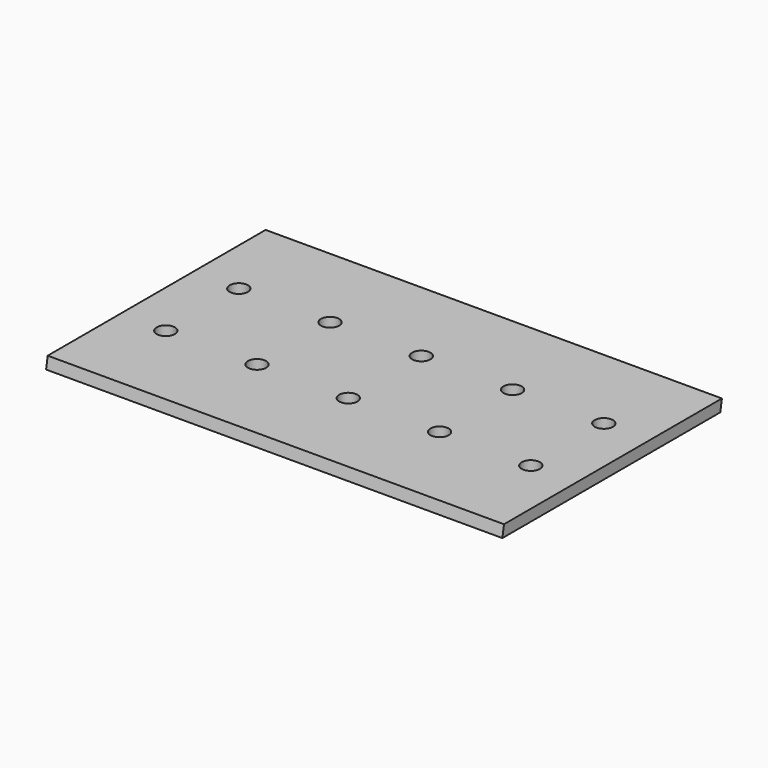
from build123d import *

# Parameters (mm, degrees)
F0_W     = 254
F0_H     = 165.1
F0_R     = 5.08
F1_DEPTH = 6.35
F3_DEPTH = 254.001
F5_DEPTH = 254.001


with BuildPart() as f1:
    # F0 (on Top) → F1 (new body)
    with BuildSketch(Plane.XY):
        with Locations((127, 82.55)):
            Rectangle(F0_W, F0_H)
        with Locations((25.4, 63.881)):
            Circle(F0_R, mode=Mode.SUBTRACT)
        with Locations((76.2, 63.881)):
            Circle(F0_R, mode=Mode.SUBTRACT)
        with Locations((127, 63.881)):
            Circle(F0_R, mode=Mode.SUBTRACT)
        with Locations((177.8, 63.881)):
            Circle(F0_R, mode=Mode.SUBTRACT)
        with Locations((228.6, 63.881)):
            Circle(F0_R, mode=Mode.SUBTRACT)
        with Locations((25.4, 114.681)):
            Circle(F0_R, mode=Mode.SUBTRACT)
        with Locations((76.2, 114.681)):
            Circle(F0_R, mode=Mode.SUBTRACT)
        with Locations((127, 114.681)):
            Circle(F0_R, mode=Mode.SUBTRACT)
        with Locations((177.8, 114.681)):
            Circle(F0_R, mode=Mode.SUBTRACT)
        with Locations((228.6, 114.681)):
            Circle(F0_R, mode=Mode.SUBTRACT)
    extrude(amount=F1_DEPTH)

    # F2 (on face) → F3 (cut, through all)
    with BuildSketch(Plane(origin=(0, 0, 0), x_dir=(0, -1, 0), z_dir=(-1, 0, 0))):
        Polygon((-163.9803236725, 0), (-165.1, 6.35), (-165.1, 0), align=None)
    extrude(amount=-F3_DEPTH, mode=Mode.SUBTRACT)

    # F4 (on face) → F5 (cut, through all)
    with BuildSketch(Plane(origin=(0, 0, 0), x_dir=(0, -1, 0), z_dir=(-1, 0, 0))):
        Polygon((0, 6.35), (-13.462, 6.35), (-12.3423236725, 0), (0, 0), align=None)
        Polygon((0, 0), (-12.3423236725, 0), (19.5333006358, -180.7756486286), (19.5333006358, 6.35), (0, 6.35), align=None)
    extrude(amount=-F5_DEPTH, mode=Mode.SUBTRACT)


solid = f1.part
